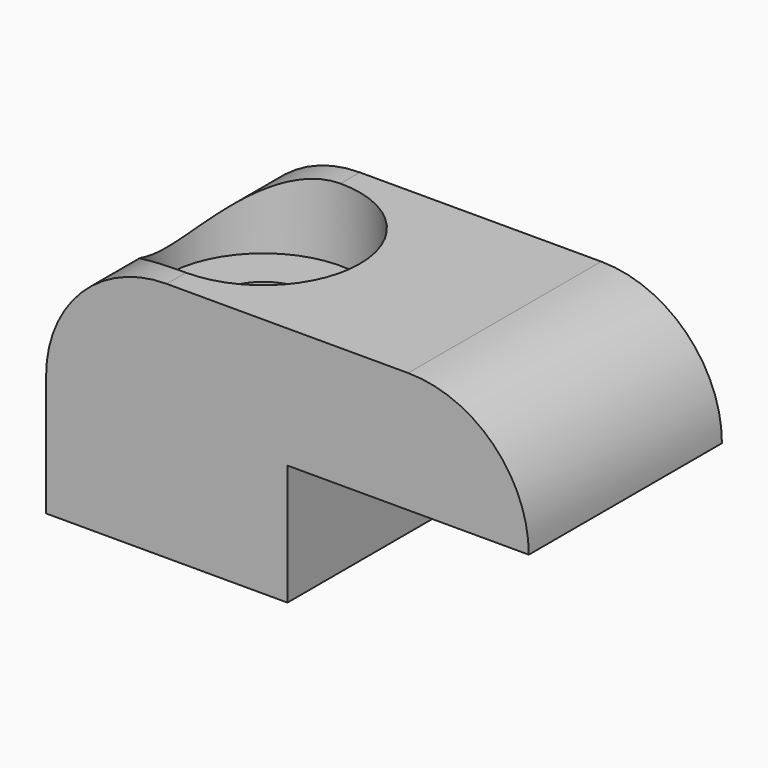
from build123d import *

# Parameters (mm, degrees)
F1_DEPTH = 10
F2_R     = 4.99999
F3_R     = 2
F4_DEPTH = 25
F5_R     = 4
F6_DEPTH = 3


# Not quite as in the source:
# - a fillet or chamfer is up to 0.001 mm smaller than in the source, because OpenCascade refuses the exact size


with BuildPart() as f1:
    # F0 (on Front) → F1 (new body)
    with BuildSketch(Plane.XZ):
        Polygon((0, 10), (0, 0), (10, 0), (10, 5), (20, 5), (20, 10), align=None)
    extrude(amount=F1_DEPTH)

    # F2 (radius 5 in the source; OpenCascade refuses exactly that, so slightly less here)
    f2_edges = [f1.edges().sort_by_distance(p)[0] for p in [
        (20, -5, 10),
        (0, -5, 10),
    ]]
    fillet(f2_edges, radius=F2_R)

    # F3 (on face) → F4 (cut)
    with BuildSketch(Plane.XY.offset(10)):
        with Locations((5, -5)):
            Circle(F3_R)
    extrude(amount=-F4_DEPTH, mode=Mode.SUBTRACT)

    # F5 (on face) → F6 (cut)
    with BuildSketch(Plane.XY.offset(10)):
        with Locations((5, -5)):
            Circle(F5_R)
    extrude(amount=-F6_DEPTH, mode=Mode.SUBTRACT)


solid = f1.part
